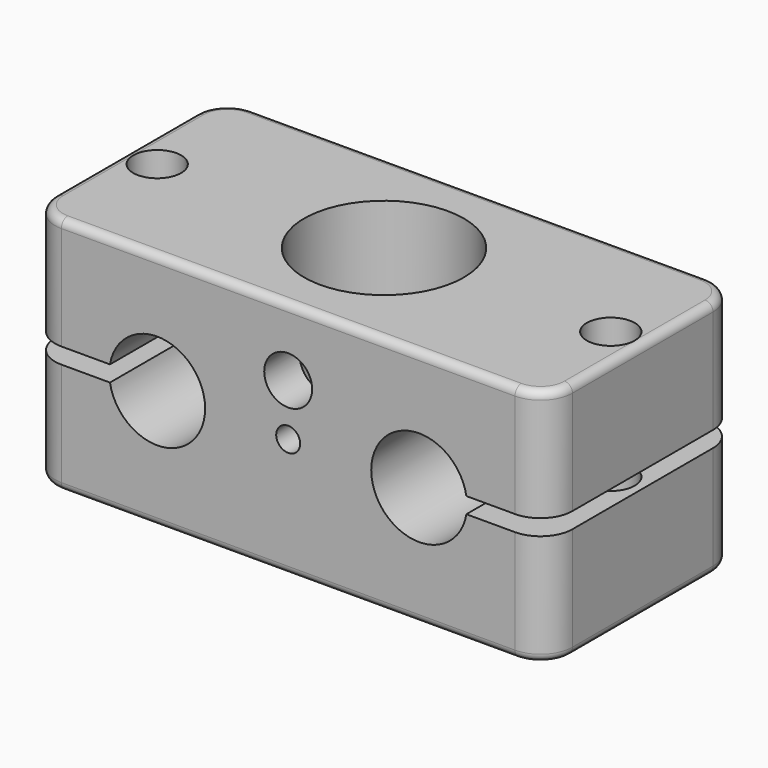
from build123d import *

# Parameters (mm, degrees)
F0_W     = 32.4
F0_H     = 15
F0_R     = 5
F1_DEPTH = 15
F3_D     = 6
F4_D     = 6
F5_DEPTH = 15
F6_DEPTH = 15
F7_D     = 3
F8_D     = 1.5
F8_DEPTH = 3
F8_TIP   = 0.4506454643
F9_D     = 3
F9_DEPTH = 3
F9_TIP   = 0.9012909285
F10_R    = 2
F11_R    = 0.49999


# Not quite as in the source:
# - a fillet or chamfer is up to 0.001 mm smaller than in the source, because OpenCascade refuses the exact size


with BuildPart() as f1:
    # F0 (on Top) → F1 (new body)
    with BuildSketch(Plane.XY):
        Rectangle(F0_W, F0_H)
        Circle(F0_R, mode=Mode.SUBTRACT)
    extrude(amount=F1_DEPTH)

    # F3 (through all)
    with Locations(Plane.XZ.offset(7.5)):
        with Locations((-8.2, 7.5)):
            Hole(F3_D / 2)

    # F4 (through all)
    with Locations(Plane.XZ.offset(7.5)):
        with Locations((8.2, 7.5)):
            Hole(F4_D / 2)

    # F2 (on face) → F5 (cut, through all)
    with BuildSketch(Plane.XZ.offset(7.5)):
        with BuildLine():
            Line((-11.1580398915, 8), (-16.2, 8))
            Line((-16.2, 8), (-16.2, 7.5))
            Line((-16.2, 7.5), (-16.2, 7))
            Line((-16.2, 7), (-11.1580398915, 7))
            ThreePointArc((-11.1580398915, 7), (-11.2, 7.5), (-11.1580398915, 8))
        make_face()
    extrude(amount=-F5_DEPTH, mode=Mode.SUBTRACT)

    # F2 (on face) → F6 (cut, through all)
    with BuildSketch(Plane.XZ.offset(7.5)):
        with BuildLine():
            ThreePointArc((11.1580398915, 8), (11.1894915684, 7.7508787808), (11.2, 7.5))
            ThreePointArc((11.2, 7.5), (11.1894915684, 7.2491212192), (11.1580398915, 7))
            Line((11.1580398915, 7), (16.2, 7))
            Line((16.2, 7), (16.2, 7.5))
            Line((16.2, 7.5), (16.2, 8))
            Line((16.2, 8), (11.1580398915, 8))
        make_face()
    extrude(amount=-F6_DEPTH, mode=Mode.SUBTRACT)

    # F7 (through all)
    with Locations(Plane(origin=(0, 0, 0), x_dir=(1, 0, 0), z_dir=(0, 0, -1))):
        with Locations((-14.2, 0), (14.2, 0)):
            Hole(F7_D / 2)

    # F8
    with Locations(Plane.XZ.offset(7.5)):
        with Locations((0, 7.5)):
            Hole(F8_D / 2, depth=F8_DEPTH)
            with Locations((0, 0, -(F8_DEPTH + F8_TIP / 2))):  # 118° drill point
                Cone(0, F8_D / 2, F8_TIP, mode=Mode.SUBTRACT)

    # F9
    with Locations(Plane.XZ.offset(7.5)):
        with Locations((0, 10.75)):
            Hole(F9_D / 2, depth=F9_DEPTH)
            with Locations((0, 0, -(F9_DEPTH + F9_TIP / 2))):  # 118° drill point
                Cone(0, F9_D / 2, F9_TIP, mode=Mode.SUBTRACT)

    # F10
    f10_edges = [f1.edges().sort_by_distance(p)[0] for p in [
        (16.2, -7.5, 11.5),
        (16.2, -7.5, 3.5),
        (16.2, 7.5, 11.5),
        (16.2, 7.5, 3.5),
        (-16.2, -7.5, 3.5),
        (-16.2, -7.5, 11.5),
        (-16.2, 7.5, 3.5),
        (-16.2, 7.5, 11.5),
    ]]
    fillet(f10_edges, radius=F10_R)

    # F11 (radius 0.5 in the source; OpenCascade refuses exactly that, so slightly less here)
    f11_edges = [f1.edges().sort_by_distance(p)[0] for p in [
        (0, -7.5, 0),
        (0, 7.5, 0),
        (0, -7.5, 15),
        (0, 7.5, 15),
    ]]
    fillet(f11_edges, radius=F11_R)


solid = f1.part
